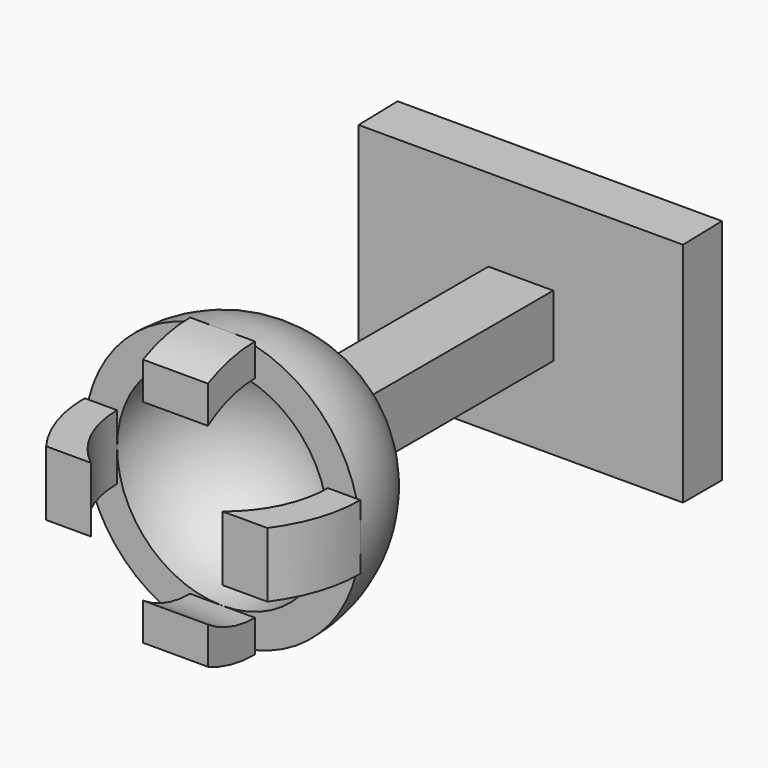
from build123d import *

# Parameters (mm, degrees)
F1_ANGLE_BACK = 90
F1_ANGLE      = 180
F3_DEPTH      = 2
F5_DEPTH      = 2
F6_W          = 15
F6_H          = 3.8226658944
F7_DEPTH      = 2
F9_DEPTH      = 10


# Not quite as in the source:
# - the program builds the solid bodies; features that only make, move or delete a surface that nothing else refers to are left out


with BuildPart() as f1:
    # F0 (on Top) → F1 (revolve)
    with BuildSketch(Plane.XY, mode=Mode.PRIVATE) as f1_sk:
        with BuildLine():
            ThreePointArc((-6.5, 0), (0, 6.5), (6.5, 0))
            Line((6.5, 0), (8.5, 0))
            ThreePointArc((8.5, 0), (0, 8.5), (-8.5, 0))
            Line((-8.5, 0), (-6.5, 0))
        make_face()
    revolve(f1_sk.sketch.rotate(Axis((7.5, 0, 0), (1, 0, 0)), -F1_ANGLE_BACK), axis=Axis((7.5, 0, 0), (1, 0, 0)), revolution_arc=F1_ANGLE)

    # F2 (on Top) → F3 (join, symmetric)
    with BuildSketch(Plane.XY):
        with BuildLine():
            Line((-6.5, 0), (-8.5, 0))
            ThreePointArc((-8.5, 0), (-8.06943757, -2.6709880764), (-6.8213700461, -5.0713815371))
            Line((-6.8213700461, -5.0713815371), (-4.0658442304, -5.0713815371))
            ThreePointArc((-4.0658442304, -5.0713815371), (-5.8599482718, -2.8126511073), (-6.5, 0))
        make_face()
        with BuildLine():
            Line((8.5, 0), (6.5, 0))
            ThreePointArc((6.5, 0), (5.8599482718, -2.8126511073), (4.0658442304, -5.0713815371))
            Line((4.0658442304, -5.0713815371), (6.8213700461, -5.0713815371))
            ThreePointArc((6.8213700461, -5.0713815371), (8.06943757, -2.6709880764), (8.5, 0))
        make_face()
    extrude(amount=F3_DEPTH, both=True)

    # F4 (on Right) → F5 (join, symmetric)
    with BuildSketch(Plane.YZ):
        with BuildLine():
            Line((0, 6.5), (0, 8.5))
            ThreePointArc((0, 8.5), (-1.8599634185, 8.2940060334), (-3.6297759564, 7.6860084898))
            Line((-3.6297759564, 7.6860084898), (-3.6297759564, 5.3920985253))
            ThreePointArc((-3.6297759564, 5.3920985253), (-1.8975457288, 6.2168577438), (0, 6.5))
        make_face()
        with BuildLine():
            Line((0, -8.5), (0, -6.5))
            ThreePointArc((0, -6.5), (-1.8975457288, -6.2168577438), (-3.6297759564, -5.3920985253))
            Line((-3.6297759564, -5.3920985253), (-3.6297759564, -7.6860084898))
            ThreePointArc((-3.6297759564, -7.6860084898), (-1.8599634185, -8.2940060334), (0, -8.5))
        make_face()
    extrude(amount=F5_DEPTH, both=True)

    # F6 (on Right) → F7 (join, symmetric)
    with BuildSketch(Plane.YZ):
        with Locations((15.7498891279, 0)):
            Rectangle(F6_W, F6_H)
    extrude(amount=F7_DEPTH, both=True)


with BuildPart() as f9:
    # F8 (on Right) → F9 (new body, symmetric)
    with BuildSketch(Plane.YZ):
        Polygon((22.991493836, 7), (22.991493836, 0), (22.991493836, -7), (25.991493836, -7), (25.991493836, 7.0670126006), align=None)
    extrude(amount=F9_DEPTH, both=True)


solid = Compound([f1.part, f9.part])
